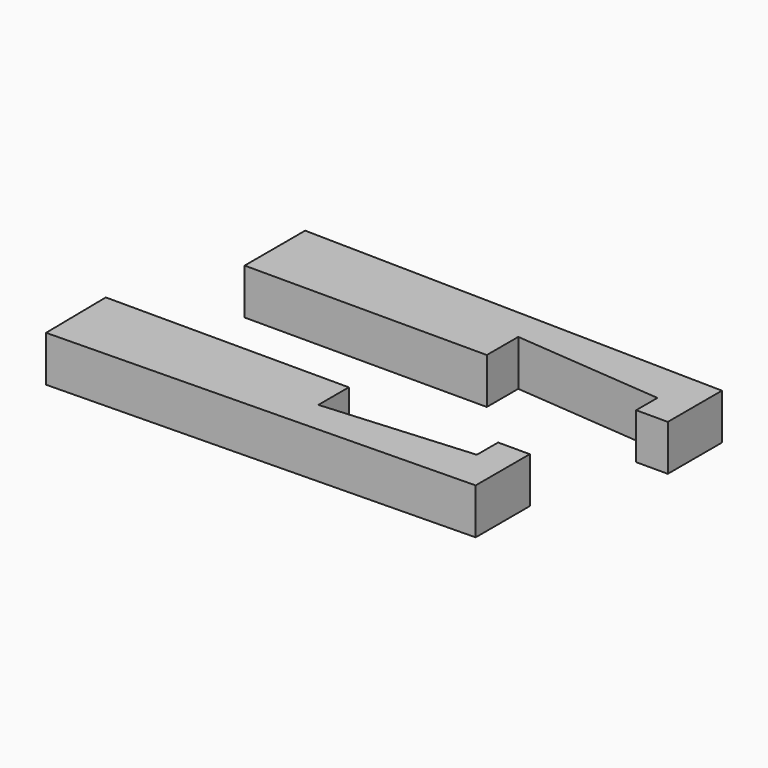
from build123d import *

# Parameters (mm, degrees)
F1_DEPTH = 5.08
F3_DEPTH = 5.08


# Not quite as in the source:
# - ends of sketch curves that miss each other by under 0.0002 mm in the source are joined


with BuildPart() as f1:
    # F0 (on Top) → F1 (new body)
    with BuildSketch(Plane.XY):
        Polygon((18.4606127441, 0), (18.4606127441, 7.51117242), (-28.5233613104, 8.40017242), (-28.5233613104, 0), (-1.6348321224, 0), (-1.6348321224, 4.1214697994), (-1.6348321224, 4.36431868), (14.9467270821, 2.9550751206), (14.9467270821, 0), align=None)
    extrude(amount=F1_DEPTH)


with BuildPart() as f3:
    # F2 (on Top) → F3 (new body)
    with BuildSketch(Plane.XY):
        Polygon((-7.1930428014, -16.4325327125), (-7.1930428014, -12.2086521793), (-34.1898388486, -12.1878198983), (-34.0815179727, -20.6088316595), (12.9024560817, -19.7198316595), (12.9024560817, -12.2086592395), (9.3885704198, -12.2086592395), (9.3885704198, -15.16373436), align=None)
    extrude(amount=F3_DEPTH)


solid = Compound([f1.part, f3.part])
